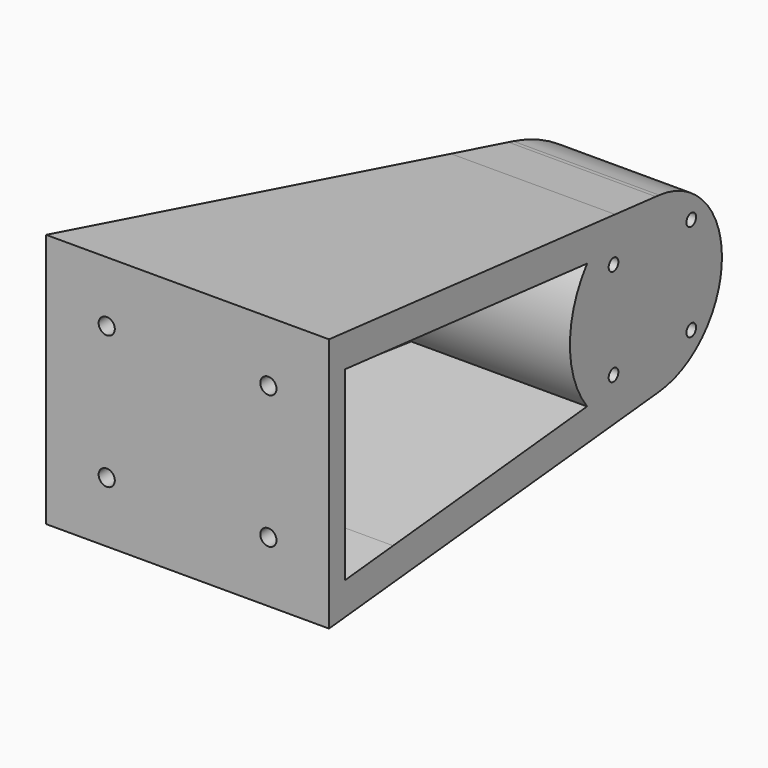
from build123d import *
from build123d import SkipClean  # not in build123d's __all__

# Parameters (mm, degrees)
F1_DEPTH = 43
F2_R     = 1.5
F3_DEPTH = 76.2
F4_REACH = 159.0367669999
F5_R     = 2
F6_DEPTH = 5
F7_START = -10
F2_R_2   = 3.6
F7_DEPTH = 40


with BuildPart() as f1:
    # F0 (on Top) → F1 (new body)
    with BuildSketch(Plane.XY):
        Polygon((17.0276526734, -48.2698833057), (17.0276526734, 72.2301166943), (-12.9723473266, 72.2301166943), (-52.9723473266, -48.2698833057), align=None)
    extrude(amount=F1_DEPTH)

    # F2 (on face) → F3 (cut)
    with BuildSketch(Plane.YZ.offset(17.0276526734)):
        with Locations((63.7509319745, 9.4791847198)):
            Circle(F2_R)
        with Locations((63.7509319745, 33.5208152802)):
            Circle(F2_R)
        with Locations((39.7093014141, 33.5208152802)):
            Circle(F2_R)
        with Locations((39.7093014141, 9.4791847198)):
            Circle(F2_R)
        with BuildLine():
            Line((72.2301166943, 36.6657508881), (72.2301166943, 43))
            Line((72.2301166943, 43), (65.4414258951, 43))
            ThreePointArc((65.4414258951, 43), (69.1264984233, 40.1444603767), (72.2301166943, 36.6657508881))
        make_face()
        with BuildLine():
            Line((72.2301166943, 0), (72.2301166943, 6.3342491119))
            ThreePointArc((72.2301166943, 6.3342491119), (69.1264984233, 2.8555396233), (65.4414258951, 0))
            Line((65.4414258951, 0), (72.2301166943, 0))
        make_face()
        with BuildLine():
            ThreePointArc((31.5312779311, 5.93539552), (26.2301166943, 21.5), (31.5312779311, 37.06460448))
            Line((31.5312779311, 37.06460448), (-28.4524949389, 43))
            Line((-28.4524949389, 43), (-43.2698833057, 43))
            Line((-43.2698833057, 43), (-43.2698833057, 0))
            Line((-43.2698833057, 0), (-28.4524949389, 0))
            Line((-28.4524949389, 0), (31.5312779311, 5.93539552))
        make_face()
        with BuildLine():
            ThreePointArc((72.2301166943, 36.6657508881), (69.1264984233, 40.1444603767), (65.4414258951, 43))
            Line((65.4414258951, 43), (52.7912383465, 43))
            Line((52.7912383465, 43), (53.8472030595, 42.8955122706))
            ThreePointArc((53.8472030595, 42.8955122706), (65.276177069, 38.1959350838), (72.2301166943, 27.9807406984))
            Line((72.2301166943, 27.9807406984), (72.2301166943, 36.6657508881))
        make_face()
        with BuildLine():
            Line((72.2301166943, 6.3342491119), (72.2301166943, 15.0192593016))
            ThreePointArc((72.2301166943, 15.0192593016), (65.276177069, 4.8040649162), (53.8472030595, 0.1044877294))
            Line((53.8472030595, 0.1044877294), (52.7912383465, 0))
            Line((52.7912383465, 0), (65.4414258951, 0))
            ThreePointArc((65.4414258951, 0), (69.1264984233, 2.8555396233), (72.2301166943, 6.3342491119))
        make_face()
    extrude(amount=-F3_DEPTH, mode=Mode.SUBTRACT)

    f4_end = Plane(origin=(-22.9147509124, 42.2786258919, 21.5), x_dir=(-0.3150460979, -0.94907637, 0), z_dir=(-0.94907637, 0.3150460979, 0))
    # F2 (on face) → F4 (join, up to a plane its end follows)
    with BuildSketch(Plane.YZ.offset(17.0276526734)):
        Polygon((-43.2698833057, 0), (-48.2698833057, 0), (-48.2698833057, -1.9609309735), (-43.2698833057, -1.466180874), align=None)
        with BuildLine():
            Line((-48.2698833057, -10), (40.2025293734, -1.2456530036))
            ThreePointArc((40.2025293734, -1.2456530036), (39.0953081378, -0.6497542366), (38.0188074935, 0))
            Line((38.0188074935, 0), (-28.4524949389, 0))
            Line((-28.4524949389, 0), (-43.2698833057, -1.466180874))
            Line((-43.2698833057, -1.466180874), (-48.2698833057, -1.9609309735))
            Line((-48.2698833057, -1.9609309735), (-48.2698833057, -10))
        make_face()
        Polygon((-43.2698833057, 44.466180874), (-48.2698833057, 44.9609309735), (-48.2698833057, 43), (-43.2698833057, 43), align=None)
        with BuildLine():
            ThreePointArc((38.0188074935, 43), (39.0953081378, 43.6497542366), (40.2025293734, 44.2456530036))
            Line((40.2025293734, 44.2456530036), (-48.2698833057, 53))
            Line((-48.2698833057, 53), (-48.2698833057, 44.9609309735))
            Line((-48.2698833057, 44.9609309735), (-43.2698833057, 44.466180874))
            Line((-43.2698833057, 44.466180874), (-28.4524949389, 43))
            Line((-28.4524949389, 43), (38.0188074935, 43))
        make_face()
        with BuildLine():
            Line((51.7301166943, 43), (52.7912383465, 43))
            Line((52.7912383465, 43), (40.2025293734, 44.2456530036))
            ThreePointArc((40.2025293734, 44.2456530036), (39.0953081378, 43.6497542366), (38.0188074935, 43))
            Line((38.0188074935, 43), (51.7301166943, 43))
        make_face()
        with BuildLine():
            Line((52.7912383465, 0), (51.7301166943, 0))
            Line((51.7301166943, 0), (38.0188074935, 0))
            ThreePointArc((38.0188074935, 0), (39.0953081378, -0.6497542366), (40.2025293734, -1.2456530036))
            Line((40.2025293734, -1.2456530036), (52.7912383465, 0))
        make_face()
        with BuildLine():
            ThreePointArc((73.2301166943, 21.5), (72.9786460552, 24.7787192622), (72.2301166943, 27.9807406984))
            Line((72.2301166943, 27.9807406984), (72.2301166943, 15.0192593016))
            ThreePointArc((72.2301166943, 15.0192593016), (72.9786460552, 18.2212807378), (73.2301166943, 21.5))
        make_face()
    f4_long = extrude(amount=-F4_REACH, mode=Mode.PRIVATE)
    add(split(f4_long, bisect_by=f4_end, keep=Keep.BOTTOM, mode=Mode.PRIVATE))

    # F5 (on face) → F6 (cut)
    with BuildSketch(Plane.XZ.offset(48.2698833057)):
        with Locations((2.0276526734, 5)):
            Circle(F5_R)
        with Locations((2.0276526734, 38)):
            Circle(F5_R)
        with Locations((-37.9723473266, 38)):
            Circle(F5_R)
        with Locations((-37.9723473266, 5)):
            Circle(F5_R)
    extrude(amount=-F6_DEPTH, mode=Mode.SUBTRACT)

    # F2 (on face) → F7 (cut)
    with BuildSketch(Plane.YZ.offset(17.0276526734).offset(F7_START)):
        with Locations((63.7509319745, 33.5208152802)):
            Circle(F2_R_2)
        with Locations((63.7509319745, 33.5208152802)):
            Circle(F2_R, mode=Mode.SUBTRACT)
        with BuildLine():
            Line((42.3226328457, 35.9967996963), (37.6318949116, 36.4609483083))
            ThreePointArc((37.6318949116, 36.4609483083), (38.0538050247, 30.3240463325), (43.3093014141, 33.5208152802))
            ThreePointArc((43.3093014141, 33.5208152802), (43.0535496969, 34.8534830644), (42.3226328457, 35.9967996963))
        make_face()
        with Locations((39.7093014141, 33.5208152802)):
            Circle(F2_R, mode=Mode.SUBTRACT)
        with BuildLine():
            ThreePointArc((42.3226328457, 35.9967996963), (40.0637902939, 37.1033196604), (37.6318949116, 36.4609483083))
            Line((37.6318949116, 36.4609483083), (42.3226328457, 35.9967996963))
        make_face()
        with BuildLine():
            Line((42.3226328457, 7.0032003037), (37.6318949116, 6.5390516917))
            ThreePointArc((37.6318949116, 6.5390516917), (40.0637902939, 5.8966803396), (42.3226328457, 7.0032003037))
        make_face()
        with BuildLine():
            ThreePointArc((43.3093014141, 9.4791847198), (38.0538050247, 12.6759536675), (37.6318949116, 6.5390516917))
            Line((37.6318949116, 6.5390516917), (42.3226328457, 7.0032003037))
            ThreePointArc((42.3226328457, 7.0032003037), (43.0535496969, 8.1465169356), (43.3093014141, 9.4791847198))
        make_face()
        with Locations((39.7093014141, 9.4791847198)):
            Circle(F2_R, mode=Mode.SUBTRACT)
        with Locations((63.7509319745, 9.4791847198)):
            Circle(F2_R_2)
        with Locations((63.7509319745, 9.4791847198)):
            Circle(F2_R, mode=Mode.SUBTRACT)
    extrude(amount=-F7_DEPTH, mode=Mode.SUBTRACT)


solid = f1.part
